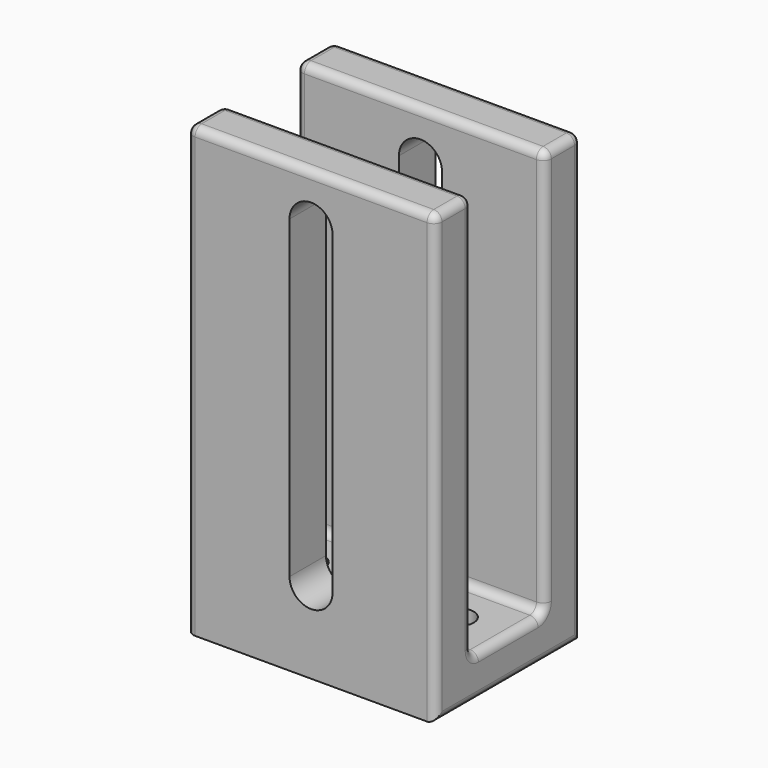
from build123d import *

# Parameters (mm, degrees)
F0_W     = 30
F0_H     = 54
F1_DEPTH = 11
F2_W     = 30
F2_H     = 11
F3_DEPTH = 49
F4_R     = 1.825
F5_DEPTH = 5
F6_F1_R  = 1
F6_F2_R  = 1


with BuildPart() as f1:
    # F0 (on Front) → F1 (new body, symmetric)
    with BuildSketch(Plane.XZ):
        with Locations((-15, 27)):
            Rectangle(F0_W, F0_H)
        with BuildLine():
            Line((-17.6, 10), (-17.6, 48))
            ThreePointArc((-17.6, 48), (-15, 50.6), (-12.4, 48))
            Line((-12.4, 48), (-12.4, 10))
            ThreePointArc((-12.4, 10), (-15, 7.4), (-17.6, 10))
        make_face(mode=Mode.SUBTRACT)
    extrude(amount=F1_DEPTH, both=True)

    # F2 (on face) → F3 (cut, through all)
    with BuildSketch(Plane.XY.offset(54)):
        with Locations((-15, 0)):
            Rectangle(F2_W, F2_H)
    extrude(amount=-F3_DEPTH, mode=Mode.SUBTRACT)

    # F4 (on Top) → F5 (cut, through all)
    with BuildSketch(Plane.XY):
        with Locations((-24, 0)):
            Circle(F4_R)
        with Locations((-6, 0)):
            Circle(F4_R)
    extrude(amount=F5_DEPTH, mode=Mode.SUBTRACT)

    # F6: fillet of radius 1 on 19 edges, made by hand

    # F6_f1
    f6_f1_edges = [f1.edges().sort_by_distance(p)[0] for p in [
        (-15, -5.5, 5),
        (-15, 5.5, 5),
    ]]
    fillet(f6_f1_edges, radius=F6_F1_R)

    # F6_f2
    f6_f2_edges = [f1.edges().sort_by_distance(p)[0] for p in [
        (-30, -11, 27),
        (-30, -5.5, 30),
        (-30, 5.5, 30),
        (0, 5.5, 30),
        (0, 11, 27),
        (-30, 11, 27),
        (-15, 11, 54),
        (-15, 5.5, 54),
        (-15, -11, 54),
        (-15, -5.5, 54),
        (0, -5.5, 30),
        (0, -11, 27),
        (0, -8.25, 54),
        (0, 8.25, 54),
        (0, 0, 0),
        (-30, -8.25, 54),
        (-30, 8.25, 54),
        (0, -5.2071067812, 5.2928932188),
        (0, 5.2071067812, 5.2928932188),
        (-30, 5.2071067812, 5.2928932188),
        (-30, -5.2071067812, 5.2928932188),
    ]]
    fillet(f6_f2_edges, radius=F6_F2_R)


solid = f1.part
